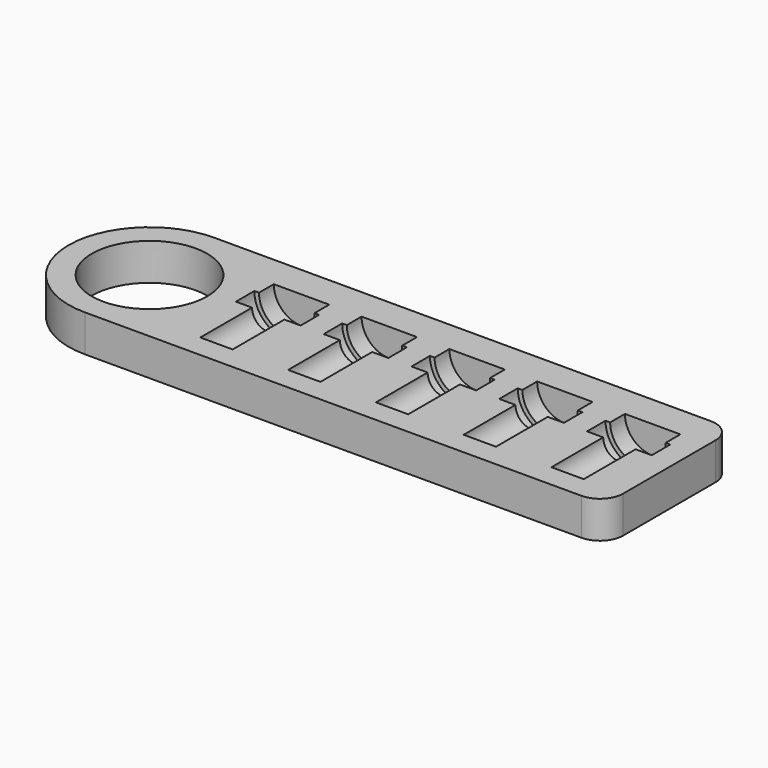
from build123d import *

# Parameters (mm, degrees)
F0_R         = 12.5
F1_DEPTH     = 8
F8_TEXT_SIZE = 5.5555555556
F9_DEPTH     = 1


# Not quite as in the source:
# - Text() gives the source's letters only with a copy of the font that has no kerning and outlines rounded to 1/6400 em; it was checked with that copy


with BuildPart() as f1:
    # F0 (on Top) → F1 (new body)
    with BuildSketch(Plane.XY):
        with BuildLine():
            ThreePointArc((0, 17.5), (5.1256313292, 5.1256313292), (17.5, 0))
            Line((17.5, 0), (125, 0))
            ThreePointArc((125, 0), (128.5355339059, 1.4644660941), (130, 5))
            Line((130, 5), (130, 30))
            ThreePointArc((130, 30), (128.5355339059, 33.5355339059), (125, 35))
            Line((125, 35), (17.5, 35))
            ThreePointArc((17.5, 35), (5.1256313292, 29.8743686708), (0, 17.5))
        make_face()
        with Locations((17.5, 17.5)):
            Circle(F0_R, mode=Mode.SUBTRACT)
    extrude(amount=F1_DEPTH)

    # F2 (on face) → F3 (revolve, cut)
    with BuildSketch(Plane.XY.offset(8)):
        Polygon((42, 19), (42, 5), (45.5, 5), (45.5, 19), (49, 19), (49, 24), (48, 24), (48, 28), (42, 28), (42, 24), align=None)
    revolve(axis=Axis((42, 21.5, 8), (0, 1, 0)), mode=Mode.SUBTRACT)

    # F2 (on face) → F4 (revolve, cut)
    with BuildSketch(Plane.XY.offset(8)):
        Polygon((61, 19), (61, 5), (64.5, 5), (64.5, 19), (68, 19), (68, 24), (67, 24), (67, 28), (61, 28), (61, 24), align=None)
    revolve(axis=Axis((61, 21.5, 8), (0, 1, 0)), mode=Mode.SUBTRACT)

    # F2 (on face) → F5 (revolve, cut)
    with BuildSketch(Plane.XY.offset(8)):
        Polygon((80, 19), (80, 5), (83.5, 5), (83.5, 19), (87, 19), (87, 24), (86, 24), (86, 28), (80, 28), (80, 24), align=None)
    revolve(axis=Axis((80, 12, 8), (0, 1, 0)), mode=Mode.SUBTRACT)

    # F2 (on face) → F6 (revolve, cut)
    with BuildSketch(Plane.XY.offset(8)):
        Polygon((99, 19), (99, 5), (102.5, 5), (102.5, 19), (106, 19), (106, 24), (105, 24), (105, 28), (99, 28), (99, 24), align=None)
    revolve(axis=Axis((99, 12, 8), (0, 1, 0)), mode=Mode.SUBTRACT)

    # F2 (on face) → F7 (revolve, cut)
    with BuildSketch(Plane.XY.offset(8)):
        Polygon((118, 19), (118, 5), (121.5, 5), (121.5, 19), (125, 19), (125, 24), (124, 24), (124, 28), (118, 28), (118, 24), align=None)
    revolve(axis=Axis((118, 12, 8), (0, 1, 0)), mode=Mode.SUBTRACT)

    # F8 (on face) → F9 (cut)
    with BuildSketch(Plane(origin=(0, 0, 0), x_dir=(1, 0, 0), z_dir=(0, 0, -1))):
        with Locations((30, -9)):
            Text('962, 1008, 1023', F8_TEXT_SIZE, font='Open Sans', text_align=(TextAlign.LEFT, TextAlign.BOTTOM))
    extrude(amount=-F9_DEPTH, mode=Mode.SUBTRACT)


solid = f1.part
